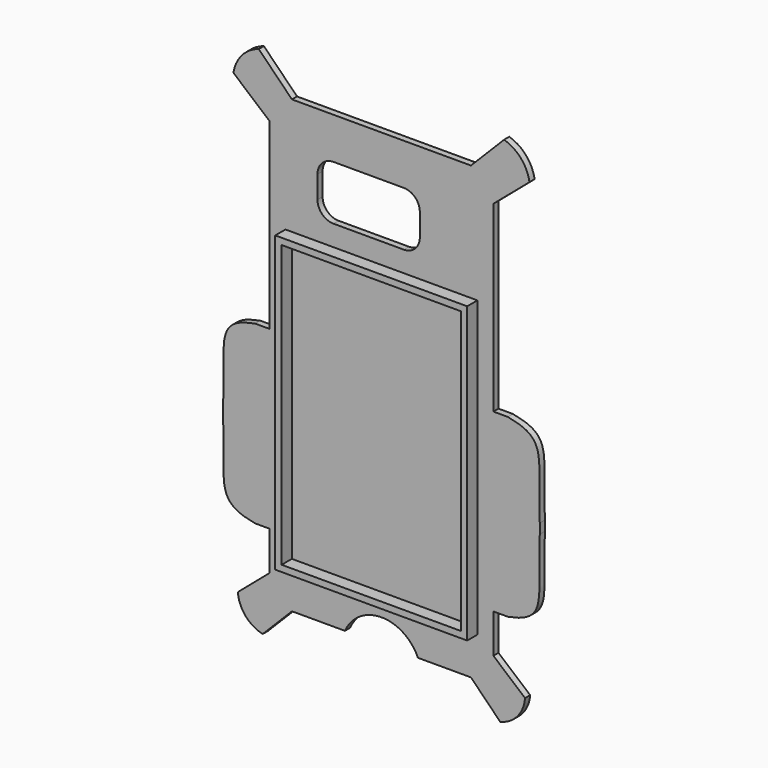
from build123d import *

# Parameters (mm, degrees)
F1_DEPTH = 2
F4_DEPTH = 3
F6_DEPTH = 4


# Not quite as in the source:
# - a feature names something its author has since deleted; it is built from what else it names


with BuildPart() as f1:
    # F0 (on Front) → F1 (new body)
    with BuildSketch(Plane.XZ):
        with BuildLine():
            Line((35, 5), (35, 62.2008182108))
            Line((35, 62.2008182108), (46.2846243068, 71.8236053681))
            ThreePointArc((46.2846243068, 71.8236053681), (43.6200052332, 77.5075823048), (38.3557090366, 80.9273738449))
            Line((38.3557090366, 80.9273738449), (27.9797695779, 70.4399573502))
            Line((27.9797695779, 70.4399573502), (-27.9797695779, 70.4399573502))
            Line((-27.9797695779, 70.4399573502), (-38.3557090366, 80.9273738449))
            ThreePointArc((-38.3557090366, 80.9273738449), (-43.6200052332, 77.5075823048), (-46.2846243068, 71.8236053681))
            Line((-46.2846243068, 71.8236053681), (-35, 62.2008182108))
            Line((-35, 62.2008182108), (-35, 5))
            Line((-35, 5), (-39.5, 5))
            add(Edge.make_bspline(
                [(-39.5, 5), (-52.1831149682, 2.6601287536), (-48.8236770034, -2.5189926382), (-49.5, -20.9609586745)],
                knots=[0, 0, 0, 0, 27.820341035, 27.820341035, 27.820341035, 27.820341035], degree=3))
            Line((-49.5, -20.9609586745), (-49.5, -24.0390413254))
            add(Edge.make_bspline(
                [(-39.5, -50), (-52.1831149682, -47.6601287536), (-48.8236770034, -42.4810073618), (-49.5, -24.0390413254)],
                knots=[0, 0, 0, 0, 27.820341035, 27.820341035, 27.820341035, 27.820341035], degree=3))
            Line((-39.5, -50), (-35, -50))
            Line((-35, -50), (-35, -62.2008182108))
            Line((-35, -62.2008182108), (-44.8918512807, -70.6359399196))
            ThreePointArc((-44.8918512807, -70.6359399196), (-42.5030006526, -76.443198976), (-37.1229104696, -79.6813303345))
            Line((-37.1229104696, -79.6813303345), (-27.9797695779, -70.4399573502))
            Line((-27.9797695779, -70.4399573502), (-11.4183901742, -70.4399573502))
            ThreePointArc((-11.4183901742, -70.4399573502), (0, -62.9893172158), (11.4183901742, -70.4399573502))
            Line((11.4183901742, -70.4399573502), (27.9797695779, -70.4399573502))
            Line((27.9797695779, -70.4399573502), (37.1229104696, -79.6813303345))
            ThreePointArc((37.1229104696, -79.6813303345), (42.5030006526, -76.443198976), (44.8918512807, -70.6359399196))
            Line((44.8918512807, -70.6359399196), (35, -62.2008182108))
            Line((35, -62.2008182108), (35, -50))
            Line((35, -50), (39.5, -50))
            add(Edge.make_bspline(
                [(39.5, -50), (52.1831149682, -47.6601287536), (48.8236770034, -42.4810073618), (49.5, -24.0390413254)],
                knots=[0, 0, 0, 0, 27.820341035, 27.820341035, 27.820341035, 27.820341035], degree=3))
            Line((49.5, -24.0390413254), (49.5, -20.9609586746))
            add(Edge.make_bspline(
                [(39.5, 5), (52.1831149682, 2.6601287536), (48.8236770034, -2.5189926382), (49.5, -20.9609586746)],
                knots=[0, 0, 0, 0, 27.820341035, 27.820341035, 27.820341035, 27.820341035], degree=3))
            Line((39.5, 5), (35, 5))
        make_face()
    extrude(amount=F1_DEPTH)

    # F3 (on offset) → F4 (cut)
    with BuildSketch(Plane.XZ.offset(2)):
        with BuildLine():
            ThreePointArc((12, 52.460730496), (10.5355339059, 55.9962644019), (7, 57.460730496))
            Line((7, 57.460730496), (-15, 57.460730496))
            ThreePointArc((-15, 57.460730496), (-18.5355339059, 55.9962644019), (-20, 52.460730496))
            Line((-20, 52.460730496), (-20, 45.460730496))
            ThreePointArc((-20, 45.460730496), (-18.5355339059, 41.9251965901), (-15, 40.460730496))
            Line((-15, 40.460730496), (7, 40.460730496))
            ThreePointArc((7, 40.460730496), (10.5355339059, 41.9251965901), (12, 45.460730496))
            Line((12, 45.460730496), (12, 52.460730496))
        make_face()
    extrude(amount=-F4_DEPTH, mode=Mode.SUBTRACT)


with BuildPart() as f6:
    # F5 (on offset) → F6 (new body)
    with BuildSketch(Plane.XZ.offset(2)):
        Polygon((-8.6902184412, 33.9803936929), (-30, 33.9803936929), (-30, -58.0196063071), (-8.6902184412, -58.0196063071), (30, -58.0196063071), (30, 33.9803936929), align=None)
        Polygon((-28, -56.0196063071), (-28, 31.9803936929), (-8.6902184412, 31.9803936929), (28, 31.9803936929), (28, -56.0196063071), (-8.6902184412, -56.0196063071), align=None, mode=Mode.SUBTRACT)
    extrude(amount=F6_DEPTH)


solid = Compound([f1.part, f6.part])
